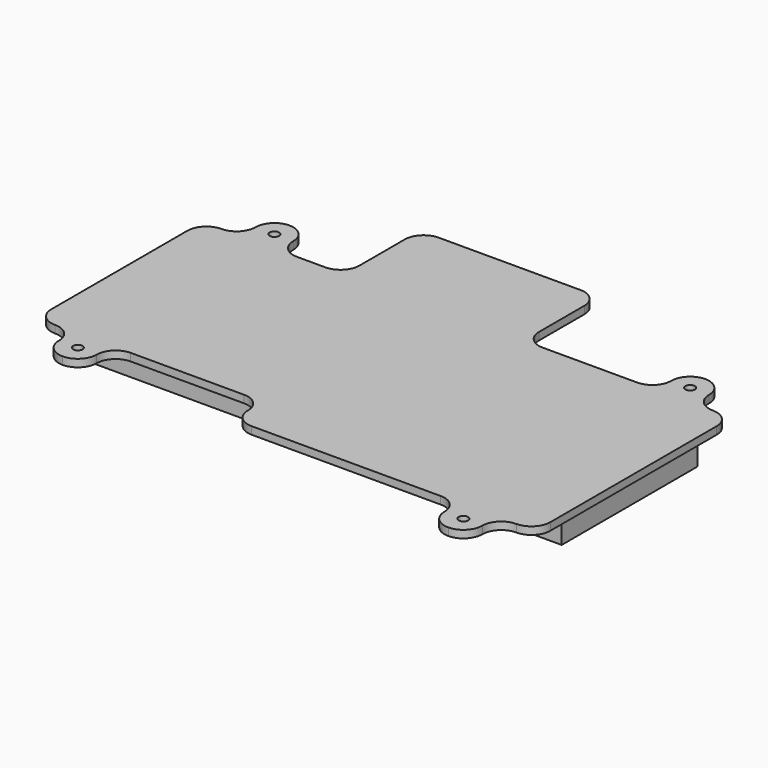
from build123d import *

# Parameters (mm, degrees)
F2_DEPTH = 2
F3_DEPTH = 9
F4_DEPTH = 5
F0_W     = 22.5
F0_H     = 25
F5_DEPTH = 18
F6_DEPTH = 7
F7_D     = 2.5


with BuildPart() as f2:
    # F1 (on Top) → F2 (new body)
    with BuildSketch(Plane.XY):
        with BuildLine():
            ThreePointArc((70, -5), (73.5355339059, -3.5355339059), (75, 0))
            Line((75, 0), (75, 55))
            ThreePointArc((75, 55), (73.5355339059, 58.5355339059), (70, 60))
            ThreePointArc((70, 60), (66.4644660941, 61.4644660941), (65, 65))
            ThreePointArc((65, 65), (63.5355339059, 68.5355339059), (60, 70))
            ThreePointArc((60, 70), (56.4644660941, 68.5355339059), (55, 65))
            ThreePointArc((55, 65), (53.5355339059, 61.4644660941), (50, 60))
            Line((50, 60), (25, 60))
            ThreePointArc((25, 60), (21.4644660941, 61.4644660941), (20, 65))
            Line((20, 65), (20, 80))
            ThreePointArc((20, 80), (18.5355339059, 83.5355339059), (15, 85))
            Line((15, 85), (-22.5, 85))
            ThreePointArc((-22.5, 85), (-26.0355339059, 83.5355339059), (-27.5, 80))
            Line((-27.5, 80), (-27.5, 65))
            ThreePointArc((-27.5, 65), (-28.9644660941, 61.4644660941), (-32.5, 60))
            Line((-32.5, 60), (-40, 60))
            ThreePointArc((-40, 60), (-43.5355339059, 61.4644660941), (-45, 65))
            ThreePointArc((-45, 65), (-46.4644660941, 68.5355339059), (-50, 70))
            ThreePointArc((-50, 70), (-53.5355339059, 68.5355339059), (-55, 65))
            ThreePointArc((-55, 65), (-56.4644660941, 61.4644660941), (-60, 60))
            ThreePointArc((-60, 60), (-63.5355339059, 58.5355339059), (-65, 55))
            Line((-65, 55), (-65, 10))
            ThreePointArc((-65, 10), (-63.5355339059, 6.4644660941), (-60, 5))
            ThreePointArc((-60, 5), (-56.4644660941, 3.5355339059), (-55, 0))
            ThreePointArc((-55, 0), (-53.5355339059, -3.5355339059), (-50, -5))
            ThreePointArc((-50, -5), (-46.4644660941, -3.5355339059), (-45, 0))
            ThreePointArc((-45, 0), (-43.5355339059, 3.5355339059), (-40, 5))
            Line((-40, 5), (-10, 5))
            ThreePointArc((-10, 5), (-6.4644660941, 3.5355339059), (-5, 0))
            ThreePointArc((-5, 0), (-3.5355339059, -3.5355339059), (0, -5))
            Line((0, -5), (50, -5))
            ThreePointArc((50, -5), (53.5355339059, -6.4644660941), (55, -10))
            ThreePointArc((55, -10), (56.4644660941, -13.5355339059), (60, -15))
            ThreePointArc((60, -15), (63.5355339059, -13.5355339059), (65, -10))
            ThreePointArc((65, -10), (66.4644660941, -6.4644660941), (70, -5))
        make_face()
        Polygon((-22.5, 55), (-22.5, 80), (15, 80), (15, 55), (70, 55), (70, 0), (0, 0), (0, 10), (-60, 10), (-60, 55), align=None, mode=Mode.SUBTRACT)
        Polygon((15, 80), (-22.5, 80), (-22.5, 55), (-60, 55), (-60, 10), (0, 10), (0, 0), (70, 0), (70, 55), (15, 55), align=None)
    extrude(amount=F2_DEPTH)

    # F0 (on Top) → F3 (join)
    with BuildSketch(Plane.XY):
        Polygon((35, 55), (35, 10), (70, 10), (70, 55), (40, 55), align=None)
    extrude(amount=-F3_DEPTH)

    # F0 (on Top) → F4 (join)
    with BuildSketch(Plane.XY):
        Polygon((15, 40), (15, 10), (35, 10), (35, 55), (15, 55), align=None)
    extrude(amount=-F4_DEPTH)

    # F0 (on Top) → F5 (join)
    with BuildSketch(Plane.XY):
        with Locations((-11.25, 67.5)):
            Rectangle(F0_W, F0_H)
    extrude(amount=-F5_DEPTH)

    # F0 (on Top) → F6 (join)
    with BuildSketch(Plane.XY):
        Polygon((-60, 10), (0, 10), (0, 40), (0, 55), (-22.5, 55), (-60, 55), align=None)
    extrude(amount=-F6_DEPTH)

    # F7 (through all)
    with Locations(Plane(origin=(0, 0, 0), x_dir=(1, 0, 0), z_dir=(0, 0, -1))):
        with Locations((60, -65), (-50, -65), (-50, 0), (60, 10)):
            Hole(F7_D / 2)


solid = f2.part
